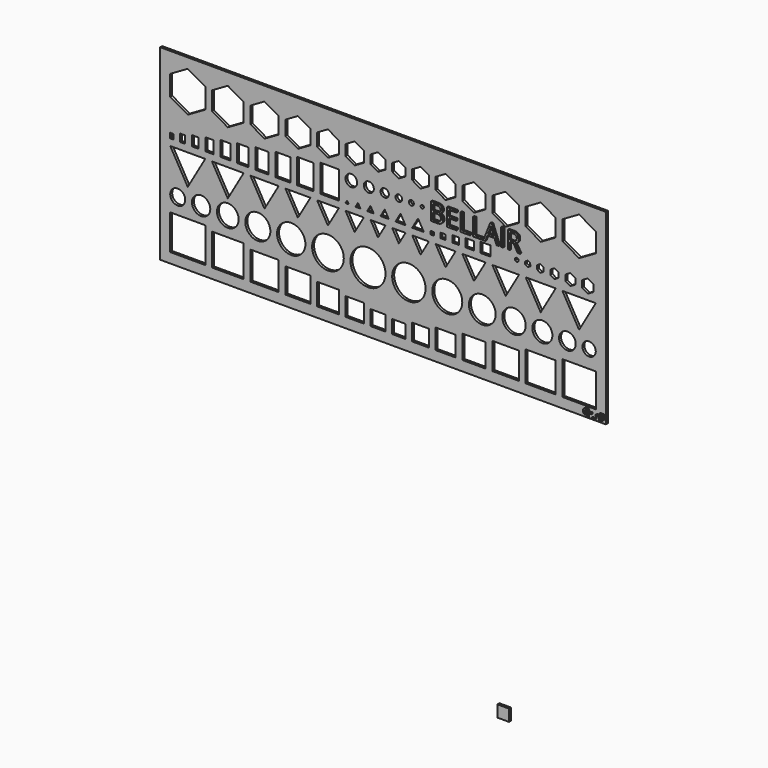
from build123d import *

# Parameters (mm, degrees)
F0_W         = 7
F0_H         = 7
F1_DEPTH     = 1.5
F0_W_2       = 267
F0_H_2       = 112.1280236695
F0_W_3       = 21
F0_H_3       = 21
F0_R         = 4.5
F0_R_2       = 5.5
F0_W_4       = 19
F0_H_4       = 19
F0_W_5       = 17
F0_H_5       = 17
F0_R_3       = 6.5
F0_R_4       = 7.5
F0_W_6       = 15
F0_H_6       = 15
F0_R_5       = 8.5
F0_W_7       = 13
F0_H_7       = 13
F0_W_8       = 11
F0_H_8       = 11
F0_W_9       = 9
F0_H_9       = 9
F0_R_6       = 9.5
F0_R_7       = 10.5
F0_W_10      = 2
F0_H_10      = 3
F0_W_11      = 3
F0_H_11      = 4.5
F0_W_12      = 4
F0_H_12      = 6
F0_W_13      = 5
F0_H_13      = 7.5
F0_W_14      = 6
F0_H_14      = 10.5
F0_W_15      = 8
F0_H_15      = 12
F0_H_16      = 13.5
F0_W_16      = 10
F0_H_17      = 16.5
F0_R_8       = 3
F0_H_18      = 8
F0_H_19      = 10
F0_R_9       = 10
F0_W_17      = 12
F0_W_18      = 14
F0_H_20      = 14
F0_R_10      = 9
F0_R_11      = 8
F0_W_19      = 16
F0_H_21      = 16
F0_W_20      = 18
F0_H_22      = 18
F0_R_12      = 7
F0_R_13      = 6
F0_W_21      = 20
F0_H_23      = 20
F0_R_14      = 5
F0_R_15      = 4
F0_H_24      = 2
F0_H_25      = 4
F0_H_26      = 5
F0_R_16      = 2.5
F0_R_17      = 2
F0_R_18      = 1.5
F0_R_19      = 1
F2_TEXT_SIZE = 14.5815519823
F3_DEPTH     = 1
F4_TEXT_SIZE = 5.6002633859
F5_DEPTH     = 1


# Not quite as in the source:
# - Text() gives the source's letters only with a copy of the font that has no kerning and outlines rounded to 1/6400 em; it was checked with that copy


with BuildPart() as f1:
    # F0 (on Front) → F1 (new body)
    with BuildSketch(Plane.XZ):
        with Locations((66.5000000737, -178.3107280108)):
            Rectangle(F0_W, F0_H)
    extrude(amount=F1_DEPTH)


with BuildPart() as f1b:
    # F0 (on Front) → F1, piece 2 (new body)
    with BuildSketch(Plane.XZ):
        with Locations((-5.5, 50.0640118348)):
            Rectangle(F0_W_2, F0_H_2)
        with Locations((-122.5, 10.5)):
            Rectangle(F0_W_3, F0_H_3, mode=Mode.SUBTRACT)
        with Locations((-128.5, 30.5)):
            Circle(F0_R, mode=Mode.SUBTRACT)
        with Locations((-114.5, 30.5)):
            Circle(F0_R_2, mode=Mode.SUBTRACT)
        with Locations((-98.5, 9.5)):
            Rectangle(F0_W_4, F0_H_4, mode=Mode.SUBTRACT)
        with Locations((-76.5, 8.5)):
            Rectangle(F0_W_5, F0_H_5, mode=Mode.SUBTRACT)
        with Locations((-98.5, 30.4999999999)):
            Circle(F0_R_3, mode=Mode.SUBTRACT)
        with Locations((-80.5, 30.4999999999)):
            Circle(F0_R_4, mode=Mode.SUBTRACT)
        with Locations((-56.5, 7.5000000003)):
            Rectangle(F0_W_6, F0_H_6, mode=Mode.SUBTRACT)
        with Locations((-60.5, 30.5)):
            Circle(F0_R_5, mode=Mode.SUBTRACT)
        with Locations((-38.5, 6.5)):
            Rectangle(F0_W_7, F0_H_7, mode=Mode.SUBTRACT)
        with Locations((-22.5, 5.5)):
            Rectangle(F0_W_8, F0_H_8, mode=Mode.SUBTRACT)
        with Locations((-8.5, 4.5)):
            Rectangle(F0_W_9, F0_H_9, mode=Mode.SUBTRACT)
        with Locations((-38.5, 30.5)):
            Circle(F0_R_6, mode=Mode.SUBTRACT)
        with Locations((-14.5, 30.5)):
            Circle(F0_R_7, mode=Mode.SUBTRACT)
        Polygon((-122.5000000002, 37.8115810376), (-133.0000000002, 55.9981145171), (-112.0000000002, 55.9981145171), align=None, mode=Mode.SUBTRACT)
        with Locations((-131.9999999263, 61.4981145171)):
            Rectangle(F0_W_10, F0_H_10, mode=Mode.SUBTRACT)
        with Locations((-125.4999999263, 62.2481145171)):
            Rectangle(F0_W_11, F0_H_11, mode=Mode.SUBTRACT)
        with Locations((-117.9999999263, 62.9981145171)):
            Rectangle(F0_W_12, F0_H_12, mode=Mode.SUBTRACT)
        with Locations((-109.4999999263, 63.7481145171)):
            Rectangle(F0_W_13, F0_H_13, mode=Mode.SUBTRACT)
        Polygon((-98.5000000002, 39.5436318452), (-108.0000000002, 55.9981145171), (-89.0000000002, 55.9981145171), align=None, mode=Mode.SUBTRACT)
        Polygon((-76.5000000002, 41.2756826531), (-85.0000000002, 55.9981145174), (-68.0000000002, 55.9981145174), align=None, mode=Mode.SUBTRACT)
        with Locations((-99.9999999263, 64.4981145171)):
            Rectangle(F0_W_14, F0_H_9, mode=Mode.SUBTRACT)
        with Locations((-89.4999999263, 65.2481145171)):
            Rectangle(F0_W, F0_H_14, mode=Mode.SUBTRACT)
        with Locations((-77.9999999263, 65.9981145171)):
            Rectangle(F0_W_15, F0_H_15, mode=Mode.SUBTRACT)
        Polygon((-122.5, 100.1280236695), (-112, 94.065845843), (-112, 81.94149019), (-122.5, 75.8793123636), (-133, 81.94149019), (-133, 94.065845843), align=None, mode=Mode.SUBTRACT)
        Polygon((-98.5, 77.0340129019), (-108, 82.5188404592), (-108, 93.4884955738), (-98.5, 98.9733231311), (-89, 93.4884955738), (-89, 82.5188404592), align=None, mode=Mode.SUBTRACT)
        Polygon((-76.5, 78.1887134403), (-85, 83.0961907284), (-85, 92.9111453047), (-76.5, 97.8186225928), (-68, 92.9111453047), (-68, 83.0961907284), align=None, mode=Mode.SUBTRACT)
        Polygon((-56.5000000002, 43.0077334606), (-64.0000000002, 55.9981145174), (-49.0000000002, 55.9981145174), align=None, mode=Mode.SUBTRACT)
        with Locations((-65.4999999263, 66.7481145171)):
            Rectangle(F0_W_9, F0_H_16, mode=Mode.SUBTRACT)
        with Locations((-51.9999999263, 67.4981145171)):
            Rectangle(F0_W_16, F0_H_6, mode=Mode.SUBTRACT)
        Polygon((-38.5000000002, 44.7397842682), (-45.0000000002, 55.9981145174), (-32.0000000002, 55.9981145174), align=None, mode=Mode.SUBTRACT)
        Polygon((-22.5000000002, 46.4718350758), (-28.0000000002, 55.9981145174), (-17.0000000002, 55.9981145174), align=None, mode=Mode.SUBTRACT)
        Polygon((-8.5000000004, 48.2038858834), (-13.0000000002, 55.9981145176), (-4.0000000002, 55.9981145174), align=None, mode=Mode.SUBTRACT)
        Polygon((-26.9999999263, 61.7301653326), (-25.9999999263, 59.9981145251), (-27.9999999263, 59.9981145251), align=None, mode=Mode.SUBTRACT)
        with Locations((-37.4999999263, 68.2481145171)):
            Rectangle(F0_W_8, F0_H_17, mode=Mode.SUBTRACT)
        Polygon((-20.4999999276, 62.5961907282), (-18.9999999263, 59.9981145176), (-21.9999999263, 59.998114516), align=None, mode=Mode.SUBTRACT)
        Polygon((-12.9999999263, 63.4622161402), (-10.9999999263, 59.9981145251), (-14.9999999263, 59.9981145251), align=None, mode=Mode.SUBTRACT)
        Polygon((-56.5, 96.6639220544), (-49, 92.3337950355), (-49, 83.6735409976), (-56.5, 79.3434139787), (-64, 83.6735409976), (-64, 92.3337950355), align=None, mode=Mode.SUBTRACT)
        with BuildLine():
            ThreePointArc((-21, 72.9981145171), (-24.5, 69.4981145171), (-28, 72.9981145171))
            ThreePointArc((-28, 72.9981145171), (-24.5, 76.4981145171), (-21, 72.9981145171))
        make_face(mode=Mode.SUBTRACT)
        Polygon((-38.5, 95.509221516), (-32, 91.7564447663), (-32, 84.2508912668), (-38.5, 80.4981145171), (-45, 84.2508912668), (-45, 91.7564447663), align=None, mode=Mode.SUBTRACT)
        Polygon((-22.5, 81.6528150555), (-28, 84.828241536), (-28, 91.1790944971), (-22.5, 94.3545209776), (-17, 91.1790944971), (-17, 84.828241536), align=None, mode=Mode.SUBTRACT)
        with Locations((-14, 72.9981145171)):
            Circle(F0_R_8, mode=Mode.SUBTRACT)
        Polygon((-8.5, 82.8075155938), (-13, 85.4055918052), (-13, 90.6017442279), (-8.5, 93.1998204392), (-4, 90.6017442279), (-4, 85.4055918052), align=None, mode=Mode.SUBTRACT)
        with Locations((4, 4)):
            Rectangle(F0_W_15, F0_H_18, mode=Mode.SUBTRACT)
        with Locations((17, 5)):
            Rectangle(F0_W_16, F0_H_19, mode=Mode.SUBTRACT)
        with Locations((10, 30.5)):
            Circle(F0_R_9, mode=Mode.SUBTRACT)
        with Locations((32, 6)):
            Rectangle(F0_W_17, F0_H_15, mode=Mode.SUBTRACT)
        with Locations((49, 7)):
            Rectangle(F0_W_18, F0_H_20, mode=Mode.SUBTRACT)
        with Locations((33, 30.5)):
            Circle(F0_R_10, mode=Mode.SUBTRACT)
        with Locations((54, 30.5)):
            Circle(F0_R_11, mode=Mode.SUBTRACT)
        with Locations((68, 8)):
            Rectangle(F0_W_19, F0_H_21, mode=Mode.SUBTRACT)
        with Locations((89, 9)):
            Rectangle(F0_W_20, F0_H_22, mode=Mode.SUBTRACT)
        with Locations((73, 30.5)):
            Circle(F0_R_12, mode=Mode.SUBTRACT)
        with Locations((90, 30.5)):
            Circle(F0_R_13, mode=Mode.SUBTRACT)
        with Locations((112, 10)):
            Rectangle(F0_W_21, F0_H_23, mode=Mode.SUBTRACT)
        with Locations((105, 30.5)):
            Circle(F0_R_14, mode=Mode.SUBTRACT)
        with Locations((118, 30.5)):
            Circle(F0_R_15, mode=Mode.SUBTRACT)
        Polygon((17, 47.3378604792), (12, 55.9981145171), (22, 55.9981145171), align=None, mode=Mode.SUBTRACT)
        Polygon((3.9999999999, 49.0699112869), (-2e-10, 55.9981145174), (8, 55.9981145174), align=None, mode=Mode.SUBTRACT)
        Polygon((-4.4999999263, 64.3282415484), (-1.9999999263, 59.9981145294), (-6.9999999263, 59.9981145294), align=None, mode=Mode.SUBTRACT)
        Polygon((5.0000000737, 65.1942669514), (8.0000000737, 59.9981145287), (2.0000000737, 59.9981145287), align=None, mode=Mode.SUBTRACT)
        with Locations((24.0000000737, 60.9981145171)):
            Rectangle(F0_W_10, F0_H_24, mode=Mode.SUBTRACT)
        Polygon((15.5000000737, 66.0602923559), (19.0000000737, 59.9981145294), (12.0000000737, 59.9981145294), align=None, mode=Mode.SUBTRACT)
        Polygon((32, 45.6058096717), (26, 55.9981145171), (38, 55.9981145171), align=None, mode=Mode.SUBTRACT)
        Polygon((49, 43.8737588641), (42, 55.9981145171), (56, 55.9981145171), align=None, mode=Mode.SUBTRACT)
        with Locations((30.5000000737, 61.4981145171)):
            Rectangle(F0_W_11, F0_H_10, mode=Mode.SUBTRACT)
        with Locations((38.0000000737, 61.9981145171)):
            Rectangle(F0_W_12, F0_H_25, mode=Mode.SUBTRACT)
        with Locations((46.5000000737, 62.4981145171)):
            Rectangle(F0_W_13, F0_H_26, mode=Mode.SUBTRACT)
        with Locations((56.0000000737, 62.9981145171)):
            Rectangle(F0_W_14, F0_H_12, mode=Mode.SUBTRACT)
        with Locations((-4.5, 72.9981145171)):
            Circle(F0_R_16, mode=Mode.SUBTRACT)
        with Locations((4, 72.9981145171)):
            Circle(F0_R_17, mode=Mode.SUBTRACT)
        Polygon((4, 83.384865863), (0, 85.6942669398), (0, 90.3130690933), (4, 92.6224701701), (8, 90.3130690933), (8, 85.6942669398), align=None, mode=Mode.SUBTRACT)
        with Locations((11.5, 72.9981145171)):
            Circle(F0_R_18, mode=Mode.SUBTRACT)
        with Locations((18, 72.9981145171)):
            Circle(F0_R_19, mode=Mode.SUBTRACT)
        Polygon((17, 93.7771707084), (22, 90.8904193625), (22, 85.1169166706), (17, 82.2301653246), (12, 85.1169166706), (12, 90.8904193625), align=None, mode=Mode.SUBTRACT)
        Polygon((32, 81.0754647863), (26, 84.5395664014), (26, 91.4677696317), (32, 94.9318712468), (38, 91.4677696317), (38, 84.5395664014), align=None, mode=Mode.SUBTRACT)
        Polygon((49, 79.9207642479), (42, 83.9622161322), (42, 92.0451199009), (49, 96.0865717852), (56, 92.0451199009), (56, 83.9622161322), align=None, mode=Mode.SUBTRACT)
        Polygon((68, 42.1417080565), (60, 55.9981145171), (76, 55.9981145171), align=None, mode=Mode.SUBTRACT)
        Polygon((89, 40.409657249), (80, 55.9981145171), (98, 55.9981145171), align=None, mode=Mode.SUBTRACT)
        Polygon((74.7341739481, 64.6528143443), (75.7348142498, 64.0765745332), (75.7360960856, 62.9218747063), (74.7367376196, 62.3434146905), (73.7360973179, 62.9196545016), (73.7348154821, 64.0743543285), align=None, mode=Mode.SUBTRACT)
        Polygon((81.2335370352, 65.2301642578), (82.7344974878, 64.3658045411), (82.7364202415, 62.6337548008), (81.2373825426, 61.7660647771), (79.73642209, 62.6304244937), (79.7344993363, 64.362474234), align=None, mode=Mode.SUBTRACT)
        Polygon((88.7380280817, 61.1887148636), (86.7367474783, 62.3411944858), (86.7341838067, 64.6505941396), (88.7329007386, 65.8075141712), (90.734181342, 64.655034549), (90.7367450136, 62.3456348952), align=None, mode=Mode.SUBTRACT)
        Polygon((112, 38.6776064417), (102, 55.9981145174), (122, 55.9981145174), align=None, mode=Mode.SUBTRACT)
        Polygon((97.2322650581, 66.3848640846), (99.7338658124, 64.9442645569), (99.7370704019, 62.0575149897), (97.238674237, 60.6113649502), (94.7370734827, 62.0519644779), (94.7338688932, 64.9387140451), align=None, mode=Mode.SUBTRACT)
        Polygon((106.7316299937, 66.9622139981), (109.7335508989, 65.2334945648), (109.7373964063, 61.7693950841), (106.7393210085, 60.0340150367), (103.7374001033, 61.76273447), (103.7335545959, 65.2268339507), align=None, mode=Mode.SUBTRACT)
        Polygon((117.2309955456, 67.5395639115), (120.7332366016, 65.5227245727), (120.7377230269, 61.4812751786), (117.2399683961, 59.4566651233), (113.73772734, 61.4735044621), (113.7332409148, 65.5149538562), align=None, mode=Mode.SUBTRACT)
        Polygon((68, 78.7660637095), (60, 83.384865863), (60, 92.6224701701), (68, 97.2412723236), (76, 92.6224701701), (76, 83.384865863), align=None, mode=Mode.SUBTRACT)
        Polygon((89, 77.6113631711), (80, 82.8075155938), (80, 93.1998204392), (89, 98.395972862), (98, 93.1998204392), (98, 82.8075155938), align=None, mode=Mode.SUBTRACT)
        Polygon((112, 76.4566626327), (102, 82.2301653246), (102, 93.7771707084), (112, 99.5506734003), (122, 93.7771707084), (122, 82.2301653246), align=None, mode=Mode.SUBTRACT)
    extrude(amount=F1_DEPTH)

    # F2 (on face) → F3 (join)
    with BuildSketch(Plane.XZ.offset(1.5)):
        with Locations((22.6940829307, 67.9160133004)):
            Text('BELLAIR', F2_TEXT_SIZE, font='Open Sans', text_align=(TextAlign.LEFT, TextAlign.BOTTOM))
    extrude(amount=F3_DEPTH)

    # F4 (on face) → F5 (join)
    with BuildSketch(Plane.XZ.offset(1.5)):
        with Locations((114.8945086359, -4.0321896378)):
            Text('q-_-p', F4_TEXT_SIZE, font='Open Sans', font_style=FontStyle.BOLD, text_align=(TextAlign.LEFT, TextAlign.BOTTOM))
    extrude(amount=F5_DEPTH)


solid = Compound([f1.part, f1b.part])
